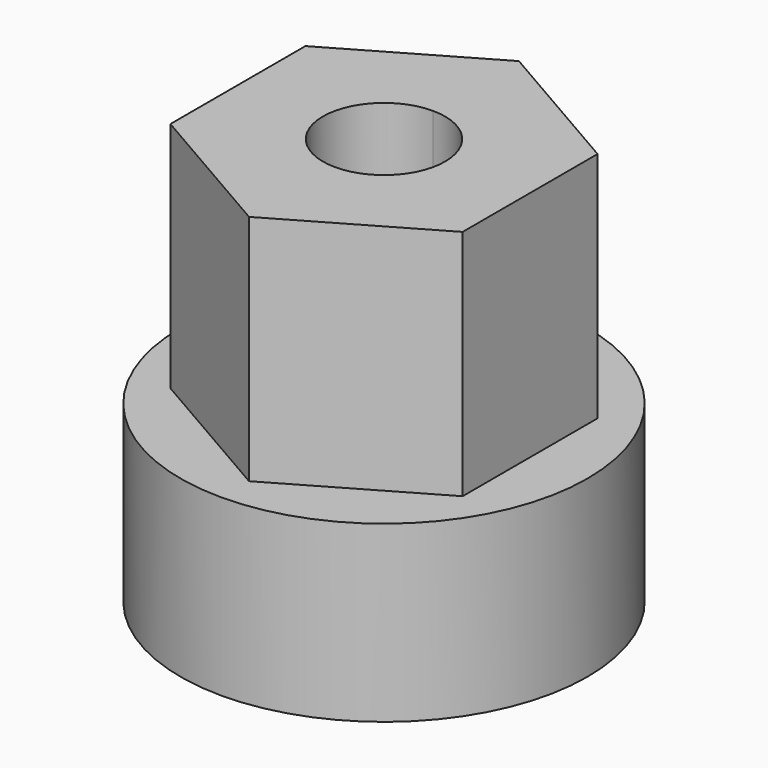
from build123d import *

# Parameters (mm, degrees)
F1_DEPTH = 4
F2_R     = 3.5
F2_R_2   = 1.05
F3_DEPTH = 3


with BuildPart() as f1:
    # F0 (on Top) → F1 (new body)
    with BuildSketch(Plane.XY):
        with BuildLine():
            Line((2.511473671, -1.45), (2.511473671, 1.45))
            Line((2.511473671, 1.45), (0, 2.9))
            Line((0, 2.9), (0, 1.05))
            ThreePointArc((0, 1.05), (0.7424621202, 0.7424621202), (1.05, 0))
            ThreePointArc((1.05, 0), (0.7424621202, -0.7424621202), (0, -1.05))
            Line((0, -1.05), (0, -2.9))
            Line((0, -2.9), (2.511473671, -1.45))
        make_face()
        with BuildLine():
            Line((0, 1.05), (0, 2.9))
            Line((0, 2.9), (-2.511473671, 1.45))
            Line((-2.511473671, 1.45), (-2.511473671, -1.45))
            Line((-2.511473671, -1.45), (0, -2.9))
            Line((0, -2.9), (0, -1.05))
            ThreePointArc((0, -1.05), (-1.05, 0), (0, 1.05))
        make_face()
    extrude(amount=F1_DEPTH)

    # F2 (on face) → F3 (join)
    with BuildSketch(Plane(origin=(0, 0, 0), x_dir=(1, 0, 0), z_dir=(0, 0, -1))):
        Circle(F2_R)
        Polygon((0, 2.9), (2.511473671, 1.45), (2.511473671, -1.45), (0, -2.9), (-2.511473671, -1.45), (-2.511473671, 1.45), align=None, mode=Mode.SUBTRACT)
        Polygon((2.511473671, -1.45), (2.511473671, 1.45), (0, 2.9), (-2.511473671, 1.45), (-2.511473671, -1.45), (0, -2.9), align=None)
        Circle(F2_R_2, mode=Mode.SUBTRACT)
        Circle(F2_R_2)
    extrude(amount=F3_DEPTH)


solid = f1.part
